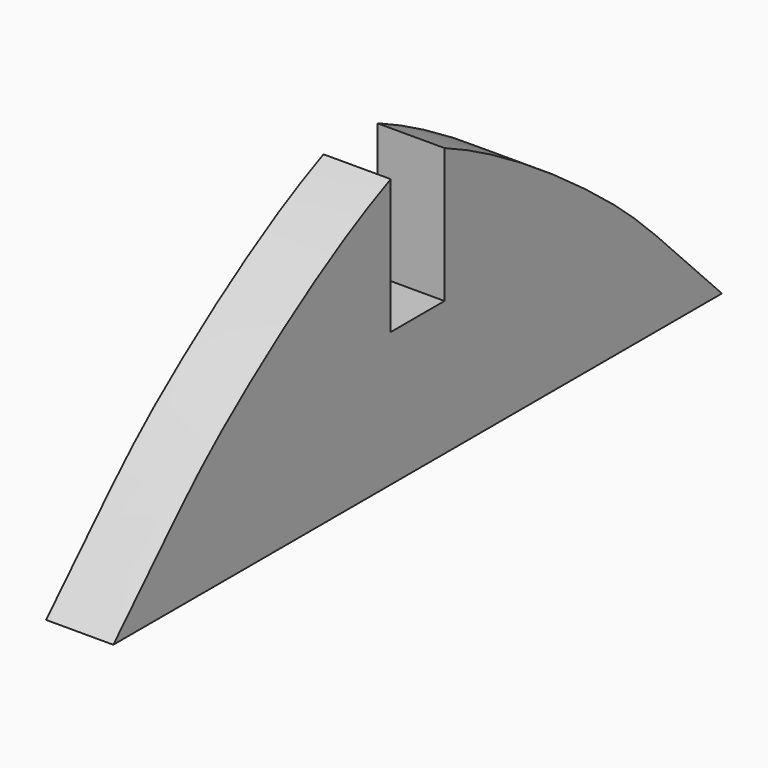
from build123d import *

# Parameters (mm, degrees)
F1_DEPTH = 38.1


with BuildPart() as f1:
    # F0 (on Right) → F1 (new body)
    with BuildSketch(Plane.YZ):
        with BuildLine():
            add(Edge.make_bspline(
                [(-132.4336230755, 0), (-83.8873000655, 49.9797638867), (-61.4657106946, 74.5330828615), (22.5918702379, 134.2773763467), (64.0371870756, 152.4)],
                knots=[0, 0, 0, 0, 0.4863937211, 1, 1, 1, 1], degree=3))
            Line((-132.4336230755, 0), (83.0871870756, 0))
            Line((83.0871870756, 0), (298.6079972267, 0))
            add(Edge.make_bspline(
                [(298.6079972267, 0), (250.0616742167, 49.9797638867), (227.6400848458, 74.5330828615), (143.5825039133, 134.2773763467), (102.1371870756, 152.4)],
                knots=[0, 0, 0, 0, 0.4863937211, 1, 1, 1, 1], degree=3))
            Line((102.1371870756, 152.4), (102.1371870756, 76.1232599616))
            Line((102.1371870756, 76.1232599616), (83.0871870756, 76.1232599616))
            Line((83.0871870756, 76.1232599616), (64.0371870756, 76.1232599616))
            Line((64.0371870756, 76.1232599616), (64.0371870756, 152.4))
        make_face()
    extrude(amount=F1_DEPTH)


solid = f1.part
